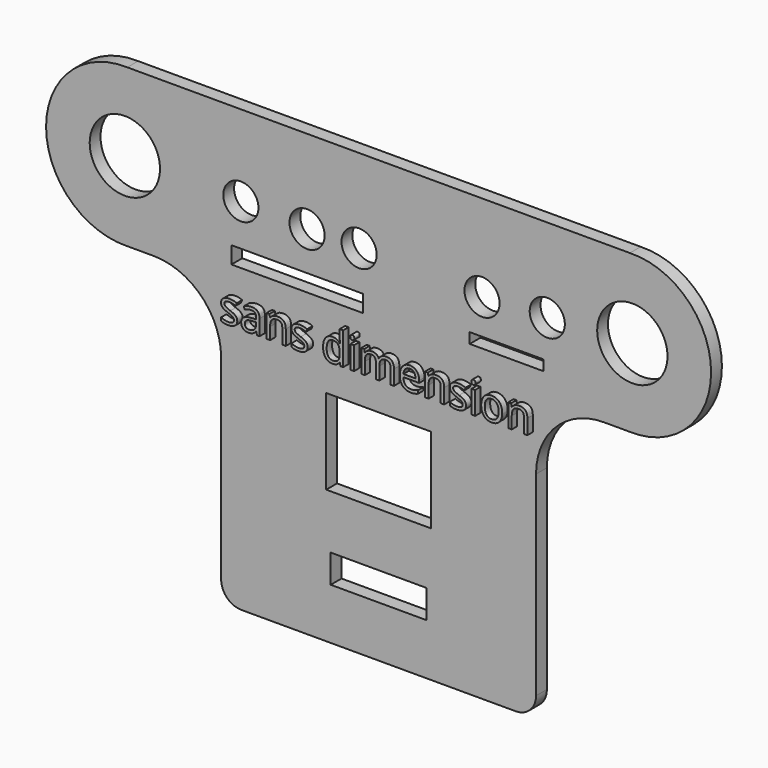
from build123d import *

# Parameters (mm, degrees)
F1_DEPTH      = 2.54
F2_R          = 12.7
F3_R          = 3.81
F6_D          = 13.2
F7_W          = 19.6568146348
F7_H          = 15.9764217678
F7_W_2        = 17.9765336215
F7_H_2        = 5.3254701197
F8_DEPTH      = 2.541
F10_D         = 6.6
F11_W         = 24.674695218
F11_H         = 3.1952820718
F11_W_2       = 13.8462316245
F11_H_2       = 1.9526742399
F12_DEPTH     = 25.4
F13_TEXT_SIZE = 8.0194996877
F14_DEPTH     = 1.27


# Not quite as in the source:
# - Text() gives the source's letters only with a copy of the font that has no kerning and outlines rounded to 1/6400 em; it was checked with that copy


with BuildPart() as f1:
    # F0 (on Front) → F1 (new body)
    with BuildSketch(Plane.XZ):
        with BuildLine():
            Line((0, -26.5704840422), (29.5559316874, -26.5704840422))
            Line((29.5559316874, -26.5704840422), (29.5559316874, 26.5704840422))
            Line((29.5559316874, 26.5704840422), (47.1700765193, 26.5704840422))
            ThreePointArc((47.1700765193, 26.5704840422), (62.414710036, 41.3484517485), (47.1700765193, 56.1264194548))
            Line((47.1700765193, 56.1264194548), (0, 56.1264194548))
            Line((0, 56.1264194548), (0, -26.5704840422))
        make_face()
    extrude(amount=F1_DEPTH)

    # F2
    f2_edges = [f1.edges().sort_by_distance(p)[0] for p in [
        (29.555932, -1.27, 26.570484),
    ]]
    fillet(f2_edges, radius=F2_R)

    # F3
    f3_edges = [f1.edges().sort_by_distance(p)[0] for p in [
        (29.555932, -1.27, -26.570484),
    ]]
    fillet(f3_edges, radius=F3_R)

    # F4: F1 across face


with BuildPart() as f1_1:
    add(f1.part)
    add(f1.part.mirror(Plane(origin=(0, -1.27, 14.7779677063), x_dir=(0, -1, 0), z_dir=(-1, 0, 0))))

    # F6 (through all)
    with Locations(Plane.XZ.offset(2.54)):
        with Locations((-47.6295995873, 41.3484517485), (47.6295995873, 41.3484517485)):
            Hole(F6_D / 2)

    # F7 (on face) → F8 (cut, through all)
    with BuildSketch(Plane.XZ.offset(2.54)):
        with Locations((0, 6.4706266858)):
            Rectangle(F7_W, F7_H)
        with Locations((0, -14.2987202853)):
            Rectangle(F7_W_2, F7_H_2)
    extrude(amount=-F8_DEPTH, mode=Mode.SUBTRACT)

    # F10 (through all)
    with Locations(Plane.XZ.offset(2.54)):
        with Locations((-25.8522666991, 40.908690542), (-13.4261623025, 40.3761416674), (-3.6627929658, 40.3761416674), (19.4142572582, 39.8435927927), (31.6628478467, 40.3761416674)):
            Hole(F10_D / 2)

    # F11 (on face) → F12 (cut)
    with BuildSketch(Plane.XZ.offset(2.54)):
        with Locations((-15.2900776593, 31.5003525466)):
            Rectangle(F11_W, F11_H)
        with Locations((24.0296693519, 32.2991739959)):
            Rectangle(F11_W_2, F11_H_2)
    extrude(amount=-F12_DEPTH, mode=Mode.SUBTRACT)

    # F13 (on face) → F14 (join)
    with BuildSketch(Plane.XZ.offset(2.54)):
        with Locations((-28.9701072033, 20.6019598991)):
            Text('sans dimension', F13_TEXT_SIZE, font='Open Sans', text_align=(TextAlign.LEFT, TextAlign.BOTTOM))
    extrude(amount=F14_DEPTH)


solid = f1_1.part
